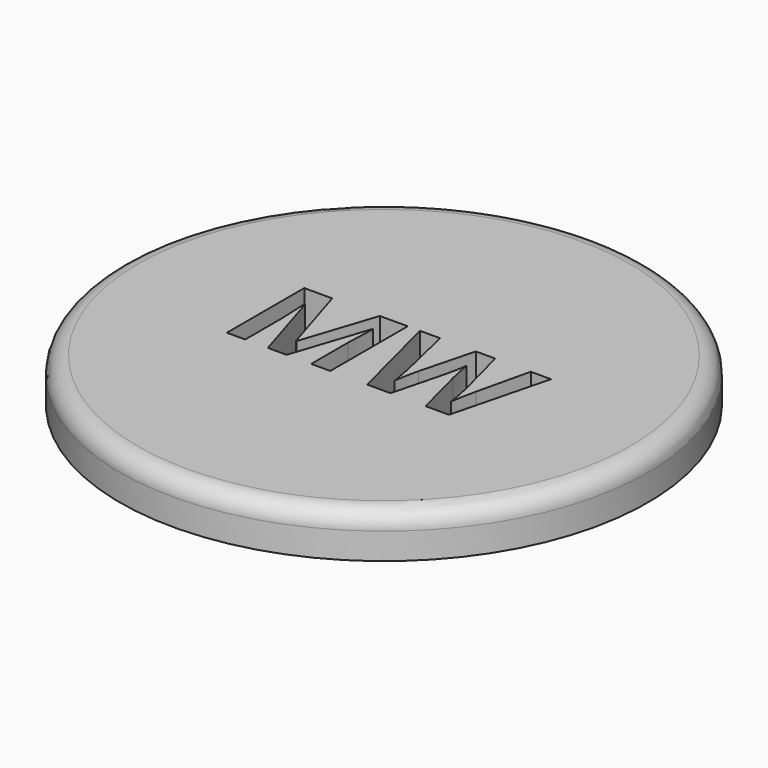
from build123d import *

# Parameters (mm, degrees)
F0_W         = 38.1
F0_H         = 6.35
F2_R         = 2.54
F3_TEXT_SIZE = 19.5691827685
F4_DEPTH     = 3.302


# Not quite as in the source:
# - Text() gives the source's letters only with a copy of the font that has no kerning and outlines rounded to 1/6400 em; it was checked with that copy


with BuildPart() as f1:
    # F0 (on Front) → F1 (revolve)
    with BuildSketch(Plane.XZ):
        with Locations((-19.05, 0)):
            Rectangle(F0_W, F0_H)
    revolve(axis=Axis((0, 0, 0), (0, 0, -1)))

    # F2
    f2_edges = [f1.edges().sort_by_distance(p)[0] for p in [
        (38.1, 0, 3.175),
    ]]
    fillet(f2_edges, radius=F2_R)

    # F3 (on Top) → F4 (cut, symmetric)
    with BuildSketch(Plane.XY):
        with Locations((-18.9960896969, -6.7933020182)):
            Text('MW', F3_TEXT_SIZE, font='Open Sans', font_style=FontStyle.BOLD, text_align=(TextAlign.LEFT, TextAlign.BOTTOM))
    extrude(amount=F4_DEPTH, both=True, mode=Mode.SUBTRACT)


solid = f1.part
